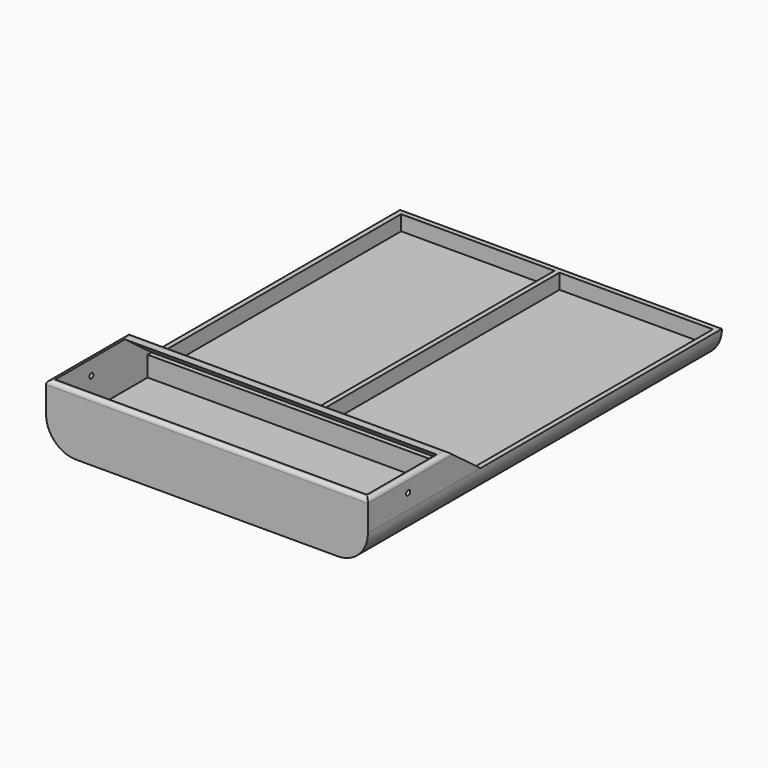
from build123d import *

# Parameters (mm, degrees)
F0_W          = 406.4
F0_H          = 558.8
F1_DEPTH      = 76.2
F3_DEPTH      = 406.4
F4_R          = 38.09999
F5_W          = 393.7
F5_H          = 374.65
F6_DEPTH      = 19.05
F8_DEPTH      = 406.4
F8_DEPTH_BACK = 6.35
F9_W          = 393.7
F9_H          = 146.05
F10_DEPTH     = 25.4
F12_DEPTH     = 6.35
F14_DEPTH     = 6.35
F15_R         = 3.175
F16_DEPTH     = 406.401
F17_R         = 5.08
F18_W         = 6.35
F18_H         = 38.1
F19_DEPTH     = 381


# Not quite as in the source:
# - a fillet or chamfer is up to 0.001 mm smaller than in the source, because OpenCascade refuses the exact size


with BuildPart() as f1:
    # F0 (on Top) → F1 (new body)
    with BuildSketch(Plane.XY):
        with Locations((-259.8249833828, -5.0296476896)):
            Rectangle(F0_W, F0_H)
    extrude(amount=F1_DEPTH)

    # F2 (on face) → F3 (cut)
    with BuildSketch(Plane(origin=(-463.0249833828, 0, 0), x_dir=(0, -1, 0), z_dir=(-1, 0, 0))):
        Polygon((5.0296476896, 76.2), (-147.3703523104, 76.2), (-96.5703523104, 38.1), (5.0296476896, 38.1), align=None)
        Polygon((157.4296476896, 76.2), (5.0296476896, 76.2), (5.0296476896, 38.1), (106.6296476896, 38.1), align=None)
        Polygon((-147.3703523104, 76.2), (-274.3703523104, 76.2), (-274.3703523104, 38.1), (-96.5703523104, 38.1), align=None)
    extrude(amount=-F3_DEPTH, mode=Mode.SUBTRACT)

    # F4 (radius 38.1 in the source; OpenCascade refuses exactly that, so slightly less here)
    f4_edges = [f1.edges().sort_by_distance(p)[0] for p in [
        (-56.624983, -5.029648, 0),
        (-463.024983, -5.029648, 0),
    ]]
    fillet(f4_edges, radius=F4_R)

    # F5 (on face) → F6 (cut)
    with BuildSketch(Plane.XY.offset(38.1)):
        with Locations((-259.8249833828, 80.6953523104)):
            Rectangle(F5_W, F5_H)
    extrude(amount=-F6_DEPTH, mode=Mode.SUBTRACT)

    # F7 (on face) → F8 (cut, two sides)
    with BuildSketch(Plane.YZ.offset(-56.6249833828)) as f8_sk:
        Polygon((-278.0796476896, 76.2), (-278.0796476896, 44.45), (-125.6796476896, 44.45), (-168.012981023, 76.2), align=None)
    extrude(amount=-F8_DEPTH, mode=Mode.SUBTRACT)
    extrude(f8_sk.sketch, amount=F8_DEPTH_BACK, mode=Mode.SUBTRACT)

    # F9 (on face) → F10 (cut)
    with BuildSketch(Plane.XY.offset(44.45)):
        with Locations((-259.8249833828, -205.0546476896)):
            Rectangle(F9_W, F9_H)
    extrude(amount=-F10_DEPTH, mode=Mode.SUBTRACT)

    # F11 (on face) → F12 (join)
    with BuildSketch(Plane.YZ.offset(-56.6249833828)):
        Polygon((-168.012981023, 76.2), (-278.0796476896, 76.2), (-278.0796476896, 44.45), (-125.6796476896, 44.45), align=None)
    extrude(amount=-F12_DEPTH)

    # F13 (on face) → F14 (join)
    with BuildSketch(Plane(origin=(-463.0249833828, 0, 0), x_dir=(0, -1, 0), z_dir=(-1, 0, 0))):
        Polygon((168.012981023, 76.2), (125.6796476896, 44.45), (278.0796476896, 44.45), (278.0796476896, 76.2), align=None)
    extrude(amount=-F14_DEPTH)

    # F15 (on face) → F16 (cut, through all)
    with BuildSketch(Plane.YZ.offset(-56.6249833828)):
        with Locations((-220.9296476896, 57.15)):
            Circle(F15_R)
    extrude(amount=-F16_DEPTH, mode=Mode.SUBTRACT)

    # F17
    f17_edges = [f1.edges().sort_by_distance(p)[0] for p in [
        (-463.024983, -220.929648, 76.2),
        (-259.824983, -157.429648, 76.2),
        (-259.824983, -284.429648, 76.2),
        (-56.624983, -220.929648, 76.2),
    ]]
    fillet(f17_edges, radius=F17_R)

    # F18 (on face) → F19 (join, through all)
    with BuildSketch(Plane(origin=(0, 274.3703523104, 0), x_dir=(-1, 0, 0), z_dir=(0, 1, 0))):
        with Locations((259.8249833828, 19.05)):
            Rectangle(F18_W, F18_H)
    extrude(amount=-F19_DEPTH)


solid = f1.part
